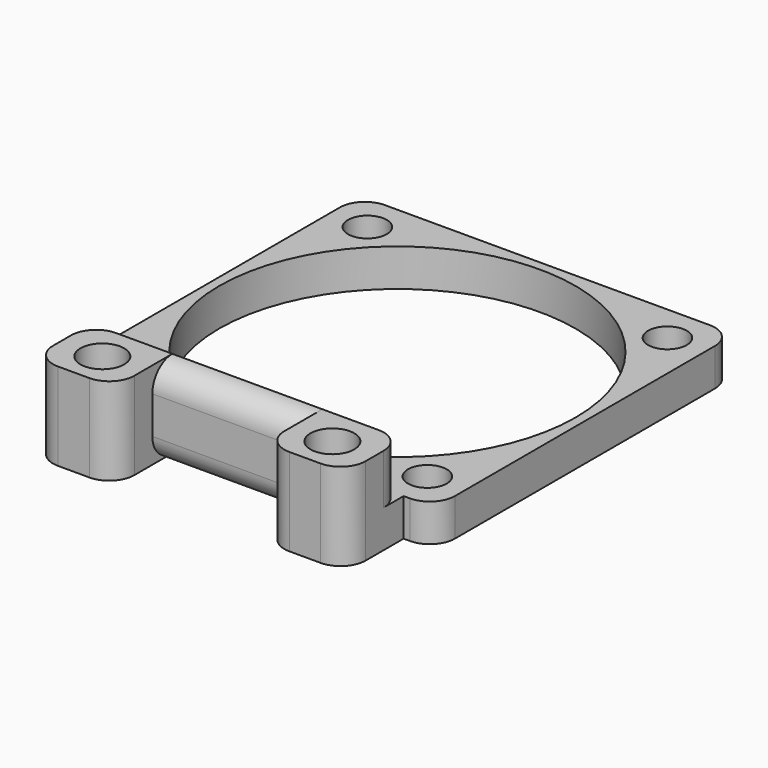
from build123d import *

# Parameters (mm, degrees)
F0_R     = 1.55
F0_R_2   = 14.25
F0_R_3   = 1.75
F0_W     = 12
F0_H     = 2
F1_DEPTH = 3
F2_DEPTH = 7
F3_R     = 2
F3_R_2   = 1.99999


# Not quite as in the source:
# - a fillet or chamfer is up to 0.001 mm smaller than in the source, because OpenCascade refuses the exact size


with BuildPart() as f1:
    # F0 (on Top) → F1 (new body)
    with BuildSketch(Plane.XY):
        Polygon((12.5, -15), (15, -15), (15, 15), (-15, 15), (-15, -15), (-12.5, -15), (-6, -15), (6, -15), align=None)
        with Locations((-12, -12)):
            Circle(F0_R, mode=Mode.SUBTRACT)
        with Locations((12, -12)):
            Circle(F0_R, mode=Mode.SUBTRACT)
        with Locations((-12, 12)):
            Circle(F0_R, mode=Mode.SUBTRACT)
        Circle(F0_R_2, mode=Mode.SUBTRACT)
        with Locations((12, 12)):
            Circle(F0_R, mode=Mode.SUBTRACT)
        Polygon((-6, -17), (-6, -15), (-12.5, -15), (-12.5, -20.8), (-6, -20.8), align=None)
        with Locations((-9.2, -18)):
            Circle(F0_R_3, mode=Mode.SUBTRACT)
        with Locations((0, -16)):
            Rectangle(F0_W, F0_H)
        Polygon((12.5, -20.8), (12.5, -15), (6, -15), (6, -17), (6, -20.8), align=None)
        with Locations((9.2, -18)):
            Circle(F0_R_3, mode=Mode.SUBTRACT)
    extrude(amount=F1_DEPTH)

    # F0 (on Top) → F2 (join)
    with BuildSketch(Plane.XY):
        with Locations((0, -16)):
            Rectangle(F0_W, F0_H)
        Polygon((-6, -17), (-6, -15), (-12.5, -15), (-12.5, -20.8), (-6, -20.8), align=None)
        with Locations((-9.2, -18)):
            Circle(F0_R_3, mode=Mode.SUBTRACT)
        Polygon((12.5, -20.8), (12.5, -15), (6, -15), (6, -17), (6, -20.8), align=None)
        with Locations((9.2, -18)):
            Circle(F0_R_3, mode=Mode.SUBTRACT)
    extrude(amount=F2_DEPTH)

    # F3 (call 1 of 12: OpenCascade refuses the feature's edges together)
    f3_edges = [f1.edges().sort_by_distance(p)[0] for p in [
        (15, -15, 1.5),
    ]]
    fillet(f3_edges, radius=F3_R)

    # F3#2 (call 2 of 12)
    f3_2_edges = [f1.edges().sort_by_distance(p)[0] for p in [
        (-15, -15, 1.5),
    ]]
    fillet(f3_2_edges, radius=F3_R)

    # F3#3 (call 3 of 12)
    f3_3_edges = [f1.edges().sort_by_distance(p)[0] for p in [
        (-15, 15, 1.5),
    ]]
    fillet(f3_3_edges, radius=F3_R)

    # F3#4 (call 4 of 12)
    f3_4_edges = [f1.edges().sort_by_distance(p)[0] for p in [
        (15, 15, 1.5),
    ]]
    fillet(f3_4_edges, radius=F3_R)

    # F3#5 (call 5 of 12)
    f3_5_edges = [f1.edges().sort_by_distance(p)[0] for p in [
        (-12.5, -20.8, 3.5),
    ]]
    fillet(f3_5_edges, radius=F3_R)

    # F3#6 (call 6 of 12)
    f3_6_edges = [f1.edges().sort_by_distance(p)[0] for p in [
        (-6, -20.8, 3.5),
    ]]
    fillet(f3_6_edges, radius=F3_R)

    # F3#7 (call 7 of 12)
    f3_7_edges = [f1.edges().sort_by_distance(p)[0] for p in [
        (6, -20.8, 3.5),
    ]]
    fillet(f3_7_edges, radius=F3_R)

    # F3#8 (call 8 of 12)
    f3_8_edges = [f1.edges().sort_by_distance(p)[0] for p in [
        (12.5, -20.8, 3.5),
    ]]
    fillet(f3_8_edges, radius=F3_R)

    # F3#9 (call 9 of 12)
    f3_9_edges = [f1.edges().sort_by_distance(p)[0] for p in [
        (12.5, -15, 5),
    ]]
    fillet(f3_9_edges, radius=F3_R)

    # F3#10 (call 10 of 12)
    f3_10_edges = [f1.edges().sort_by_distance(p)[0] for p in [
        (-12.5, -15, 5),
    ]]
    fillet(f3_10_edges, radius=F3_R)

    # F3#11 (call 11 of 12) (radius 2 in the source; OpenCascade refuses exactly that, so slightly less here)
    f3_11_edges = [f1.edges().sort_by_distance(p)[0] for p in [
        (0, -17, 7),
    ]]
    fillet(f3_11_edges, radius=F3_R_2)

    # F3#12 (call 12 of 12)
    f3_12_edges = [f1.edges().sort_by_distance(p)[0] for p in [
        (0, -17, 0),
    ]]
    fillet(f3_12_edges, radius=F3_R)


solid = f1.part
